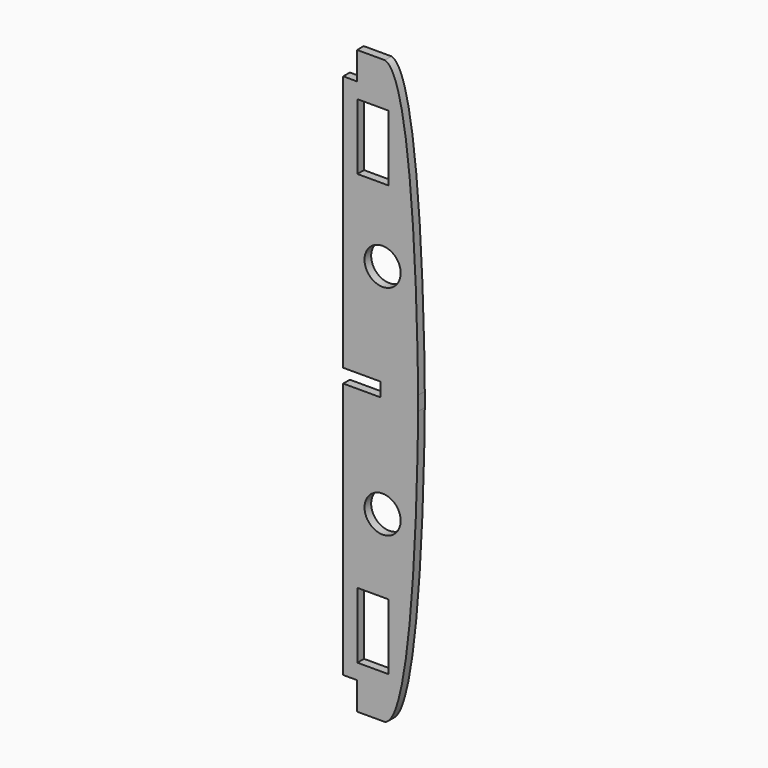
from build123d import *

# Parameters (mm, degrees)
F0_W     = 22.2654491663
F0_H     = 47.4806427956
F0_R     = 13.033720186
F1_DEPTH = 6


# Not quite as in the source:
# - a feature names something its author has since deleted; it is built from what else it names


with BuildPart() as f1:
    # F0 (on Front) → F1 (new body)
    with BuildSketch(Plane.XZ):
        with BuildLine():
            add(Edge.make_bspline(
                [(111.8640829768, 215), (133.0716213469, 209.4330211779), (135.6474762559, 42.6029998371), (135.8640829768, 10.1536091521)],
                knots=[0, 0, 0, 0, 186.7738886147, 186.7738886147, 186.7738886147, 186.7738886147], degree=3))
            Line((111.8640829768, 215), (91.8640829768, 215))
            Line((91.8640829768, 215), (91.8640829768, 195))
            Line((91.8640829768, 195), (81.8640829768, 195))
            Line((81.8640829768, 195), (81.8640829768, 10))
            Line((81.8640829768, 10), (108.8640829768, 10))
            Line((108.8640829768, 10), (108.8640829768, 5))
            Line((108.8640829768, 5), (135.8640829768, 5))
            Line((135.8640829768, 5), (135.8640829768, 10.1536091521))
        make_face()
        with Locations((103.1980912897, 160.0865775181)):
            Rectangle(F0_W, F0_H, mode=Mode.SUBTRACT)
        with Locations((110.2482031796, 83.6049893333)):
            Circle(F0_R, mode=Mode.SUBTRACT)
        with BuildLine():
            Line((135.8640829768, -0.1536091521), (135.8640829768, 5))
            Line((135.8640829768, 5), (108.8640829768, 5))
            Line((108.8640829768, 5), (108.8640829768, 0))
            Line((108.8640829768, 0), (81.8640829768, 0))
            Line((81.8640829768, 0), (81.8640829768, -185))
            Line((81.8640829768, -185), (91.8640829768, -185))
            Line((91.8640829768, -185), (91.8640829768, -205))
            Line((91.8640829768, -205), (111.8640829768, -205))
            add(Edge.make_bspline(
                [(111.8640829768, -205), (133.0716213469, -199.4330211779), (135.6474762559, -32.6029998371), (135.8640829768, -0.1536091521)],
                knots=[0, 0, 0, 0, 186.7738886147, 186.7738886147, 186.7738886147, 186.7738886147], degree=3))
        make_face()
        with Locations((103.1980912897, -150.0865775181)):
            Rectangle(F0_W, F0_H, mode=Mode.SUBTRACT)
        with Locations((110.2482031796, -73.6049893333)):
            Circle(F0_R, mode=Mode.SUBTRACT)
    extrude(amount=F1_DEPTH)


solid = f1.part
